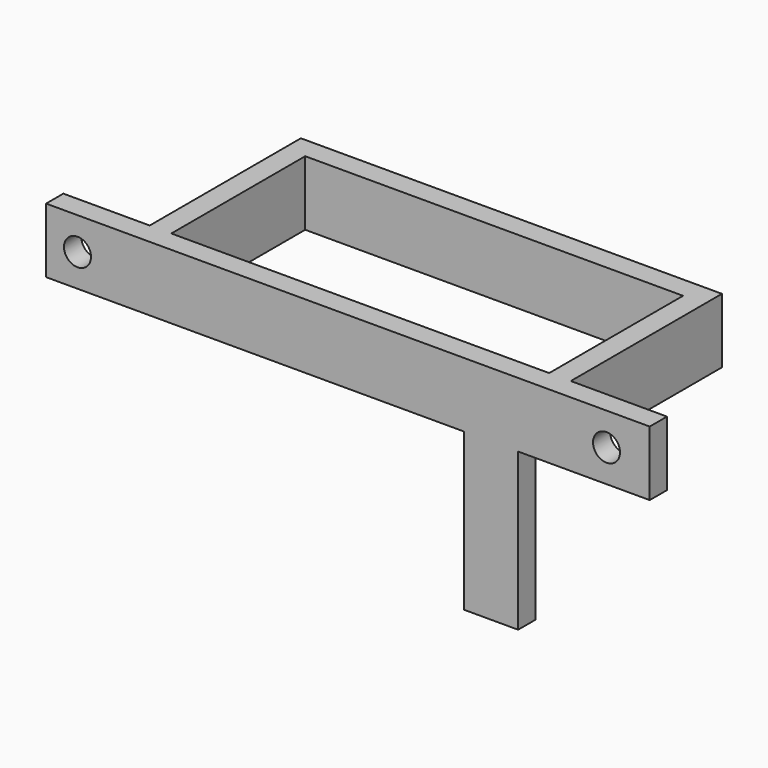
from build123d import *

# Parameters (mm, degrees)
F0_W     = 35
F0_H     = 15.5
F1_DEPTH = 3
F2_R     = 1.25
F3_DEPTH = 12.5
F5_DEPTH = 2


# Not quite as in the source:
# - a feature names something its author has since deleted; it is built from what else it names


with BuildPart() as f1:
    # F0 (on Top) → F1 (new body, symmetric)
    with BuildSketch(Plane.XY):
        Polygon((-49, 0), (-57, 0), (-57, -2), (-1.0886418074, -2), (-1.0886418074, 0), (-10, 0), (-10, 17.5), (-49, 17.5), align=None)
        with Locations((-29.5, 7.75)):
            Rectangle(F0_W, F0_H, mode=Mode.SUBTRACT)
    extrude(amount=F1_DEPTH, both=True)

    # F2 (on face) → F3 (cut, symmetric)
    with BuildSketch(Plane.XZ.offset(2)):
        with Locations((-54.0886418074, 0)):
            Circle(F2_R)
        with Locations((-5.0886418074, 0)):
            Circle(F2_R)
    extrude(amount=F3_DEPTH, both=True, mode=Mode.SUBTRACT)

    # F4 (on Front) → F5 (join)
    with BuildSketch(Plane.XZ):
        Polygon((-13.2752051018, -17.5318677962), (-13.2752051018, -2.6883990917), (-18.2752051018, -2.6883990917), (-18.2752051018, -3.858309805), (-18.2752051018, -17.5318677962), align=None)
    extrude(amount=F5_DEPTH)


solid = f1.part
